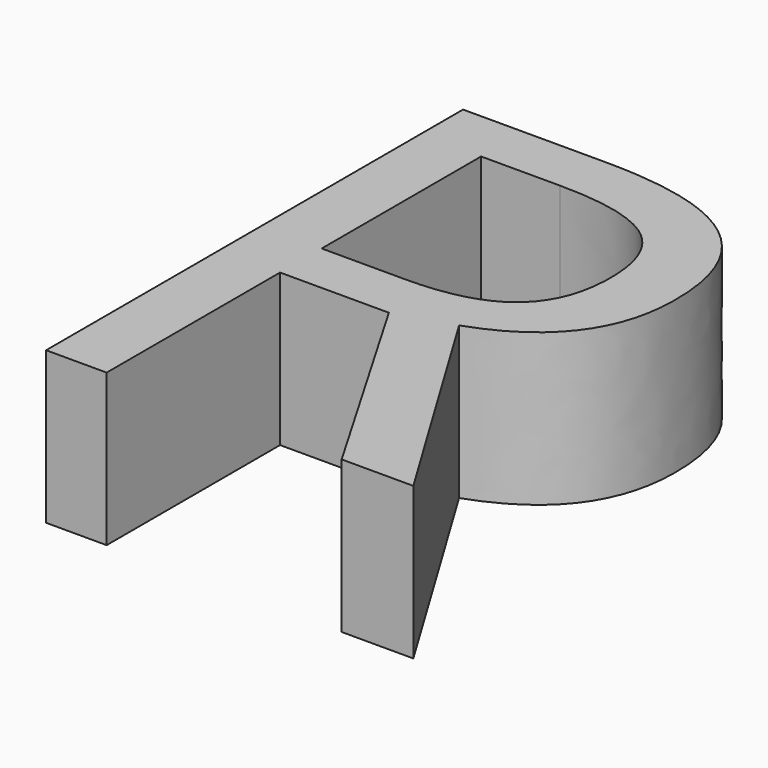
from build123d import *

# Parameters (mm, degrees)
F0_TEXT_SIZE = 120.1313937119
F1_DEPTH     = 25
F2_R         = 1.5875
F3_DEPTH     = 12.5


# Not quite as in the source:
# - Text() gives the source's letters only with a copy of the font that has no kerning and outlines rounded to 1/6400 em; it was checked with that copy


with BuildPart() as f1:
    # F0 (on Top) → F1 (new body)
    with BuildSketch(Plane.XY):
        with Locations((-34.1426085471, -49.2791602925)):
            Text('R', F0_TEXT_SIZE, font='Open Sans', text_align=(TextAlign.LEFT, TextAlign.BOTTOM))
    extrude(amount=F1_DEPTH)

    # F2 (on face) → F3 (cut)
    with BuildSketch(Plane(origin=(0, 0, 0), x_dir=(1, 0, 0), z_dir=(0, 0, -1))):
        with Locations((-17.3711397531, 29.9150943756)):
            Circle(F2_R)
        with Locations((20.4056631774, 29.9150943756)):
            Circle(F2_R)
        with Locations((-17.3711397531, -19.8113229126)):
            Circle(F2_R)
    extrude(amount=-F3_DEPTH, mode=Mode.SUBTRACT)


solid = f1.part
